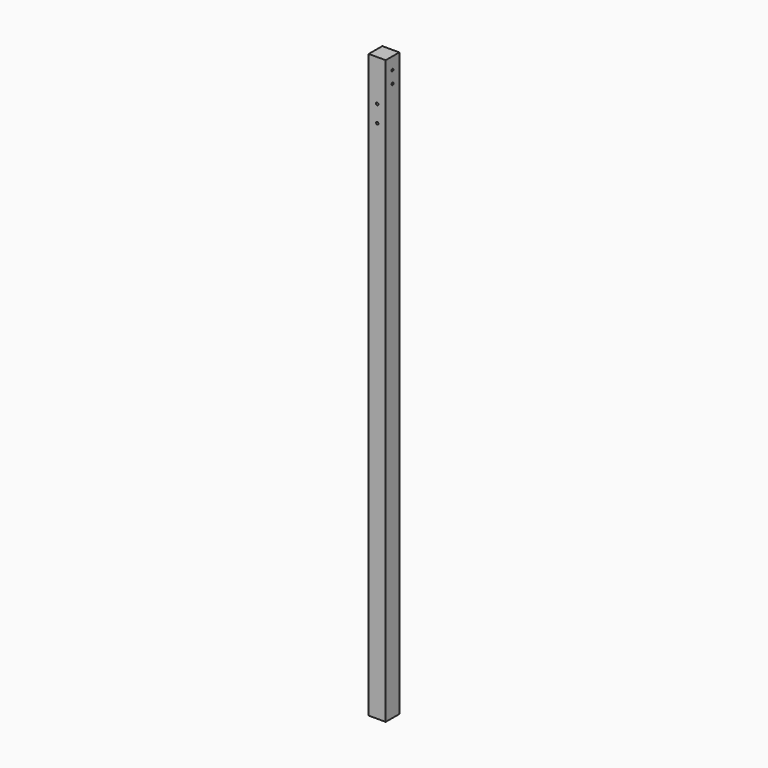
from build123d import *

# Parameters (mm, degrees)
F0_W     = 88.9
F0_H     = 3048
F1_DEPTH = 88.9
F3_D     = 12.7
F5_D     = 12.7


# Not quite as in the source:
# - a length typed as a fraction of an inch, garbled in the dataset ("3 / 203.2 mm" for 3/8 in), is restored


with BuildPart() as f1:
    # F0 (on Front) → F1 (new body)
    with BuildSketch(Plane.XZ):
        with Locations((44.45, -1524)):
            Rectangle(F0_W, F0_H)
    extrude(amount=F1_DEPTH)

    # F3 (through all)
    with Locations(Plane.XZ.offset(88.9)):
        with Locations((44.45, -215.9), (44.45, -304.8)):
            Hole(F3_D / 2)

    # F5 (through all)
    with Locations(Plane(origin=(0, 0, 0), x_dir=(0, -1, 0), z_dir=(-1, 0, 0))):
        with Locations((44.45, -63.5), (44.45, -127)):
            Hole(F5_D / 2)


solid = f1.part
